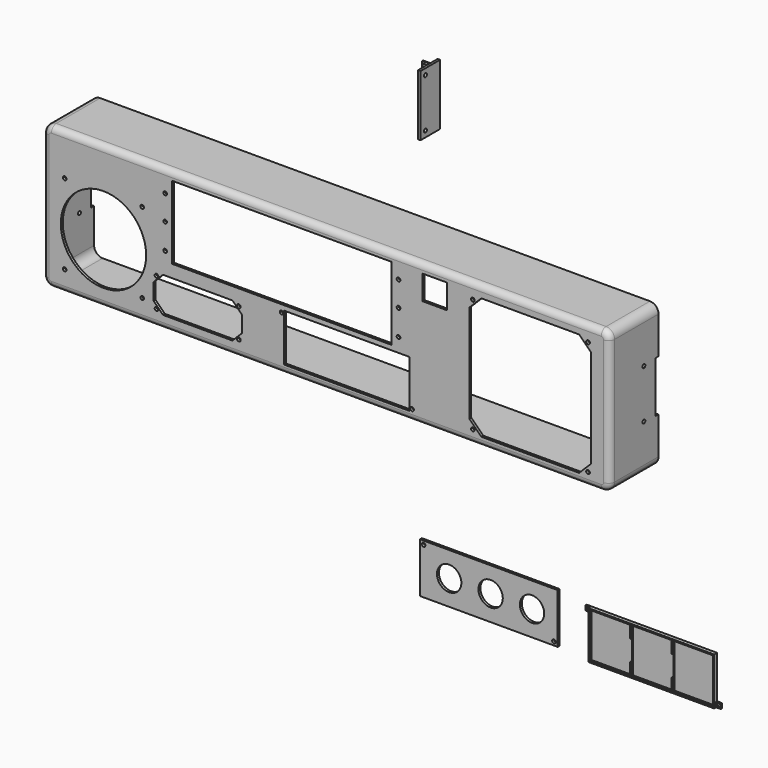
from build123d import *

# Parameters (mm, degrees)
F0_W            = 465
F0_H            = 117
F1_DEPTH        = 50
F2_T            = -2
F4_R            = 7
F3_W            = 180
F3_H            = 60
F3_W_2          = 20
F3_H_2          = 20
F3_R            = 1.5
F3_W_3          = 93
F3_H_3          = 36
F3_R_2          = 9.5
F3_R_3          = 35
F3_W_4          = 103
F3_H_4          = 39
F5_DEPTH        = 25
F6_R            = 5
F8_R            = 1.5
F8_W            = 3
F8_H            = 42
F9_DEPTH        = 500
F10_W           = 20
F10_H           = 50
F10_R           = 1.5
F11_DEPTH       = 2
F12_W           = 12
F12_H           = 40
F13_DEPTH       = 2
F15_D           = 3
F15_CSINK_D     = 5.7
F15_CSINK_ANGLE = 90
F16_SIZE        = 1
F17_W           = 113
F17_H           = 41
F17_R           = 1.5
F17_R_2         = 10
F18_DEPTH       = 2
F20_DEPTH       = 3
F19_W           = 4
F19_H           = 4
F19_R           = 1.5
F21_DEPTH       = 1
F23_DEPTH       = 2
F22_W           = 1
F22_H           = 17
F24_DEPTH       = 3


with BuildPart() as f1:
    # F0 (on Front) → F1 (new body)
    with BuildSketch(Plane.XZ):
        with Locations((-12.6529467106, 27.1878533959)):
            Rectangle(F0_W, F0_H)
    extrude(amount=F1_DEPTH)

    # F2
    f2_openings = [f1.faces().sort_by_distance(p)[0] for p in [
        (-12.652947, 0, 27.187853),
    ]]
    offset(amount=F2_T, openings=f2_openings)

    # F4
    f4_edges = [f1.edges().sort_by_distance(p)[0] for p in [
        (-245.152947, -25, 85.687853),
        (219.847053, -25, 85.687853),
        (219.847053, -25, -31.312147),
        (-245.152947, -25, -31.312147),
        (-243.152947, -24, 83.687853),
        (-243.152947, -24, -29.312147),
        (217.847053, -24, -29.312147),
        (217.847053, -24, 83.687853),
    ]]
    fillet(f4_edges, radius=F4_R)

    # F3 (on face) → F5 (cut)
    with BuildSketch(Plane.XZ.offset(50)):
        with Locations((-49.312419115, 48.5197262004)):
            Rectangle(F3_W, F3_H)
        with Locations((76.3836680665, 68.3190373614)):
            Rectangle(F3_W_2, F3_H_2)
        Polygon((194.7213235501, 76.111191912), (114.5203134233, 76.111191912), (104.6208184867, 66.2116969754), (104.6208184867, -13.9893131514), (114.5203134233, -23.888808088), (194.7213235501, -23.888808088), (204.6208184867, -13.9893131514), (204.6208184867, 66.2116969754), align=None)
        with Locations((46.5855184052, 67.5480939005)):
            Circle(F3_R)
        with Locations((46.5855184052, 47.158148972)):
            Circle(F3_R)
        with Locations((46.5855184052, 26.052269754)):
            Circle(F3_R)
        with Locations((107.5167332374, 72.8625404379)):
            Circle(F3_R)
        with Locations((93.1539236558, -72.7683771119)):
            Rectangle(F3_W_3, F3_H_3)
        with Locations((63.5958272868, -74.4846176776)):
            Circle(F3_R_2, mode=Mode.SUBTRACT)
        with Locations((93.6227975534, -74.4846176776)):
            Circle(F3_R_2, mode=Mode.SUBTRACT)
        with Locations((50.6539236558, -58.7683771119)):
            Circle(F3_R, mode=Mode.SUBTRACT)
        with Locations((135.6539236558, -86.7683771119)):
            Circle(F3_R, mode=Mode.SUBTRACT)
        with Locations((123.0111705607, -74.4846176776)):
            Circle(F3_R_2, mode=Mode.SUBTRACT)
        Polygon((-89.7012186204, 8.1878533959), (-146.7012186204, 8.1878533959), (-154.4793932134, 0.4096788029), (-154.4793932134, -13.033972011), (-146.7012186204, -20.8121466041), (-89.7012186204, -20.8121466041), (-81.9230440273, -13.033972011), (-81.9230440273, 0.4096788029), align=None)
        with Locations((-151.9793932134, 5.6878533959)):
            Circle(F3_R)
        with Locations((-151.9793932134, -18.3121466041)):
            Circle(F3_R)
        with Locations((-84.4230440273, 5.6878533959)):
            Circle(F3_R)
        with Locations((-84.4230440273, -18.3121466041)):
            Circle(F3_R)
        with Locations((107.5167332374, -20.8455865502)):
            Circle(F3_R)
        with Locations((202.0370356229, -20.8455660029)):
            Circle(F3_R)
        with Locations((202.0370356229, 72.8625404379)):
            Circle(F3_R)
        with Locations((-195.4793932134, 17.7347333959)):
            Circle(F3_R_3)
        with Locations((-144.8539147958, 67.5480939005)):
            Circle(F3_R)
        with Locations((-144.8539147958, 47.158148972)):
            Circle(F3_R)
        with Locations((-144.8539147958, 26.052269754)):
            Circle(F3_R)
        with Locations((-227.2830040105, 51.6578833959)):
            Circle(F3_R)
        with Locations((-227.2830040105, -14.1012566041)):
            Circle(F3_R)
        with Locations((-163.6415483004, -14.1012566041)):
            Circle(F3_R)
        with Locations((-163.6757824164, 51.6578833959)):
            Circle(F3_R)
        with Locations((-49.3271809206, 12.611191912)):
            Circle(F3_R)
        with Locations((57.6728190794, -22.388808088)):
            Circle(F3_R)
        with Locations((4.1728190794, -4.888808088)):
            Rectangle(F3_W_4, F3_H_4)
    extrude(amount=-F5_DEPTH, mode=Mode.SUBTRACT)

    # F6
    f6_edges = [f1.edges().sort_by_distance(p)[0] for p in [
        (217.796801, -50, 83.637601),
    ]]
    fillet(f6_edges, radius=F6_R)

    # F8 (on face) → F9 (cut)
    with BuildSketch(Plane(origin=(-245.1529467106, 0, 0), x_dir=(0, -1, 0), z_dir=(-1, 0, 0))):
        with Locations((15, 47.1878533959)):
            Circle(F8_R)
        with Locations((15, 7.1878533959)):
            Circle(F8_R)
        with Locations((1.5, 27.1878533959)):
            Rectangle(F8_W, F8_H)
    extrude(amount=-F9_DEPTH, mode=Mode.SUBTRACT)


with BuildPart() as f11:
    # F10 (on Right) → F11 (new body)
    with BuildSketch(Plane.YZ):
        with Locations((38.3660052121, 146.8174463511)):
            Rectangle(F10_W, F10_H)
        with Locations((33.3660052121, 126.8174463511)):
            Circle(F10_R, mode=Mode.SUBTRACT)
        with Locations((33.3660052121, 166.8174463511)):
            Circle(F10_R, mode=Mode.SUBTRACT)
    extrude(amount=F11_DEPTH)

    # F12 (on face) → F13 (join)
    with BuildSketch(Plane(origin=(0, 48.3660052121, 0), x_dir=(-1, 0, 0), z_dir=(0, 1, 0))):
        with Locations((6, 146.8174463511)):
            Rectangle(F12_W, F12_H)
    extrude(amount=-F13_DEPTH)

    # F15 (through all)
    with Locations(Plane.XZ.offset(-46.3660052121)):
        with Locations((-7, 156.8174463511), (-7, 136.8174463511)):
            CounterSinkHole(F15_D / 2, F15_CSINK_D / 2, counter_sink_angle=F15_CSINK_ANGLE)

    # F16
    f16_edges = [f11.edges().sort_by_distance(p)[0] for p in [
        (-6, 46.366005, 166.817446),
        (-12, 46.366005, 146.817446),
        (-6, 46.366005, 126.817446),
    ]]
    chamfer(f16_edges, length=F16_SIZE)


with BuildPart() as f18:
    # F17 (on Front) → F18 (new body)
    with BuildSketch(Plane.XZ):
        with Locations((82.2173821926, -166.7715502977)):
            Rectangle(F17_W, F17_H)
        with Locations((135.7173821926, -184.2715502977)):
            Circle(F17_R, mode=Mode.SUBTRACT)
        with Locations((49.7173821926, -166.7715502977)):
            Circle(F17_R_2, mode=Mode.SUBTRACT)
        with Locations((28.7173821926, -149.2715502977)):
            Circle(F17_R, mode=Mode.SUBTRACT)
        with Locations((83.7173821926, -166.7715502977)):
            Circle(F17_R_2, mode=Mode.SUBTRACT)
        with Locations((117.7173821926, -166.7715502977)):
            Circle(F17_R_2, mode=Mode.SUBTRACT)
    extrude(amount=F18_DEPTH)


with BuildPart() as f20:
    # F19 (on Front) → F20 (new body)
    with BuildSketch(Plane.XZ):
        Polygon((267.8700156212, -150.314532876), (164.8700156212, -150.314532876), (164.8700156212, -154.314532876), (164.8700156212, -189.314532876), (267.8700156212, -189.314532876), (267.8700156212, -185.314532876), align=None)
    extrude(amount=F20_DEPTH)

    # F19 (on Front) → F21 (join)
    with BuildSketch(Plane.XZ):
        with Locations((162.8700156212, -152.314532876)):
            Rectangle(F19_W, F19_H)
        with Locations((162.8700156212, -152.314532876)):
            Circle(F19_R, mode=Mode.SUBTRACT)
        with Locations((269.8700156212, -187.314532876)):
            Rectangle(F19_W, F19_H)
        with Locations((269.8700156212, -187.314532876)):
            Circle(F19_R, mode=Mode.SUBTRACT)
    extrude(amount=F21_DEPTH)

    # F22 (on face) → F23 (cut)
    with BuildSketch(Plane.XZ.offset(3)):
        Polygon((198.8700156212, -151.314532876), (165.8700156212, -151.314532876), (165.8700156212, -188.314532876), (198.8700156212, -188.314532876), (198.8700156212, -178.314532876), (198.8700156212, -161.314532876), align=None)
        Polygon((199.8700156212, -151.314532876), (199.8700156212, -161.314532876), (199.8700156212, -178.314532876), (199.8700156212, -188.314532876), (232.8700156212, -188.314532876), (232.8700156212, -178.314532876), (232.8700156212, -161.314532876), (232.8700156212, -151.314532876), align=None)
        Polygon((233.8700156212, -151.314532876), (233.8700156212, -161.314532876), (233.8700156212, -178.314532876), (233.8700156212, -188.314532876), (266.8700156212, -188.314532876), (266.8700156212, -151.314532876), align=None)
    extrude(amount=-F23_DEPTH, mode=Mode.SUBTRACT)

    # F22 (on face) → F24 (cut)
    with BuildSketch(Plane.XZ.offset(3)):
        with Locations((199.3700156212, -169.814532876)):
            Rectangle(F22_W, F22_H)
        with Locations((233.3700156212, -169.814532876)):
            Rectangle(F22_W, F22_H)
    extrude(amount=-F24_DEPTH, mode=Mode.SUBTRACT)


solid = Compound([f1.part, f11.part, f18.part, f20.part])
